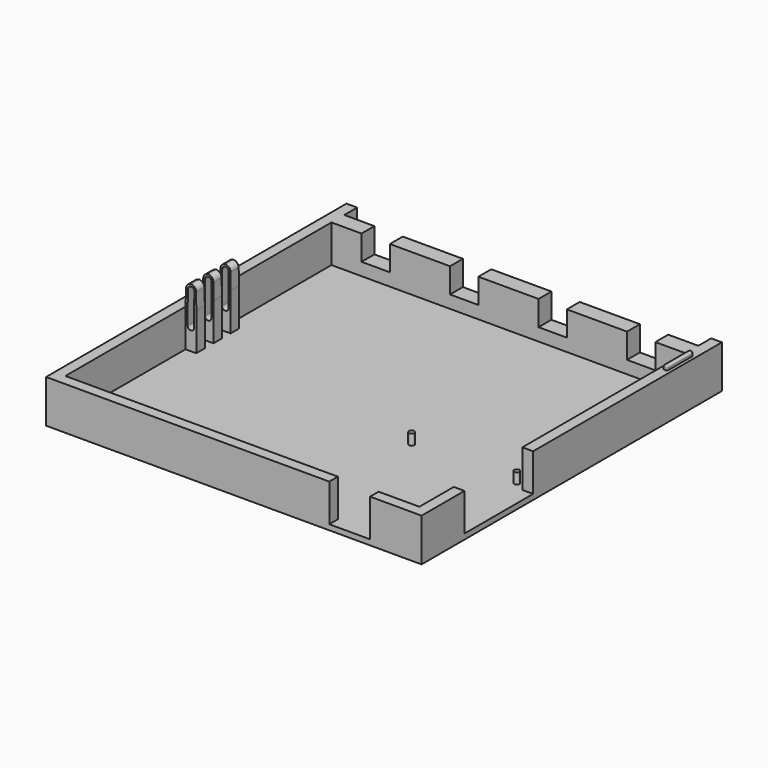
from build123d import *

# Parameters (mm, degrees)
F0_W           = 175
F0_H           = 175
F1_DEPTH       = 20
F2_W           = 165
F2_H           = 155
F3_DEPTH       = 17.5
F4_R           = 1.25
F5_DEPTH       = 5
F6_W           = 165
F6_H           = 7.5
F7_DEPTH       = 17.5
F8_W           = 13.2
F8_H           = 5.7
F9_DEPTH       = 8.5
F10_W          = 5
F10_H          = 5
F11_DEPTH      = 17.5
F11_DEPTH_BACK = 10
F11_TAPER_BACK = 1
F12_T1_DEPTH   = 16.9346144904
F12_T3_DEPTH   = 16.9346144904
F12_T5_DEPTH   = 16.9346144904
F14_DEPTH      = 25
F15_W          = 19
F15_H          = 17.6808023453
F15_W_2        = 32.2772479057
F15_H_2        = 40
F16_DEPTH      = 17.5
F17_W          = 13.2
F17_H          = 5.9
F18_DEPTH      = 8.5
F19_W          = 2
F19_H          = 15
F20_DEPTH      = 2
F21_R          = 0.99999
F22_R          = 0.5


# Not quite as in the source:
# - a fillet or chamfer that OpenCascade refuses, or shapes differently, is made with other operations: its cross-section is extruded or revolved along the edge and cut away or added
# - a fillet or chamfer is up to 0.001 mm smaller than in the source, because OpenCascade refuses the exact size


with BuildPart() as f1:
    # F0 (on Top) → F1 (new body)
    with BuildSketch(Plane.XY):
        Rectangle(F0_W, F0_H)
    extrude(amount=F1_DEPTH)

    # F2 (on face) → F3 (cut)
    with BuildSketch(Plane.XY.offset(20)):
        with Locations((0, -5)):
            Rectangle(F2_W, F2_H)
    extrude(amount=-F3_DEPTH, mode=Mode.SUBTRACT)

    # F4 (on face) → F5 (join)
    with BuildSketch(Plane.XY.offset(2.5)):
        with Locations((28.5, -77.5)):
            Circle(F4_R)
        with Locations((28.5, -19.5)):
            Circle(F4_R)
        with Locations((77.5, -77.5)):
            Circle(F4_R)
        with Locations((77.5, -19.5)):
            Circle(F4_R)
    extrude(amount=F5_DEPTH)

    # F6 (on face) → F7 (cut)
    with BuildSketch(Plane.XY.offset(20)):
        with Locations((0, 83.75)):
            Rectangle(F6_W, F6_H)
    extrude(amount=-F7_DEPTH, mode=Mode.SUBTRACT)

    # F8 (on face) → F9 (cut)
    with BuildSketch(Plane(origin=(0, 80, 0), x_dir=(-1, 0, 0), z_dir=(0, 1, 0))):
        with Locations((-61.875, 11.25)):
            Rectangle(F8_W, F8_H)
        with Locations((-20.625, 11.25)):
            Rectangle(F8_W, F8_H)
        with Locations((20.625, 11.25)):
            Rectangle(F8_W, F8_H)
        with Locations((61.875, 11.25)):
            Rectangle(F8_W, F8_H)
    extrude(amount=-F9_DEPTH, mode=Mode.SUBTRACT)

    # F10 (on face) → F11 (join, two sides)
    with BuildSketch(Plane.XY.offset(20)) as f11_sk:
        with Locations((-80, 0)):
            Rectangle(F10_W, F10_H)
        with Locations((-80, 10)):
            Rectangle(F10_W, F10_H)
        with Locations((-80, -10)):
            Rectangle(F10_W, F10_H)
    extrude(amount=-F11_DEPTH)
    extrude(f11_sk.sketch, amount=F11_DEPTH_BACK, taper=F11_TAPER_BACK)

    # F12: fillet of radius 2.5 on 6 edges, made by hand

    # F12_s2 → F12_t1 (cut)
    with BuildSketch(Plane.XZ.offset(-18.4673072452)):
        with BuildLine():
            ThreePointArc((-82.3683254308, 27.5436310161), (-81.6209793537, 29.2831261229), (-79.8687061929, 30))
            Line((-79.8687061929, 30), (-82.3254493507, 30))
            Line((-82.3254493507, 30), (-82.3683254308, 27.5436310161))
        make_face()
        with BuildLine():
            ThreePointArc((-80.1312938071, 30), (-78.3790206463, 29.2831261229), (-77.6316745692, 27.5436310161))
            Line((-77.6316745692, 27.5436310161), (-77.6745506493, 30))
            Line((-77.6745506493, 30), (-80.1312938071, 30))
        make_face()
    extrude(amount=F12_T1_DEPTH, mode=Mode.SUBTRACT)

    # F12_s4 → F12_t3 (cut)
    with BuildSketch(Plane.XZ.offset(-8.4673072452)):
        with BuildLine():
            ThreePointArc((-82.3683254308, 27.5436310161), (-81.6209793537, 29.2831261229), (-79.8687061929, 30))
            Line((-79.8687061929, 30), (-82.3254493507, 30))
            Line((-82.3254493507, 30), (-82.3683254308, 27.5436310161))
        make_face()
        with BuildLine():
            ThreePointArc((-80.1312938071, 30), (-78.3790206463, 29.2831261229), (-77.6316745692, 27.5436310161))
            Line((-77.6316745692, 27.5436310161), (-77.6745506493, 30))
            Line((-77.6745506493, 30), (-80.1312938071, 30))
        make_face()
    extrude(amount=F12_T3_DEPTH, mode=Mode.SUBTRACT)

    # F12_s6 → F12_t5 (cut)
    with BuildSketch(Plane.XZ.offset(1.5326927548)):
        with BuildLine():
            ThreePointArc((-82.3683254308, 27.5436310161), (-81.6209793537, 29.2831261229), (-79.8687061929, 30))
            Line((-79.8687061929, 30), (-82.3254493507, 30))
            Line((-82.3254493507, 30), (-82.3683254308, 27.5436310161))
        make_face()
        with BuildLine():
            ThreePointArc((-80.1312938071, 30), (-78.3790206463, 29.2831261229), (-77.6316745692, 27.5436310161))
            Line((-77.6316745692, 27.5436310161), (-77.6745506493, 30))
            Line((-77.6745506493, 30), (-80.1312938071, 30))
        make_face()
    extrude(amount=F12_T5_DEPTH, mode=Mode.SUBTRACT)

    # F13 (on face) → F14 (cut)
    with BuildSketch(Plane(origin=(0, 12.5, 0), x_dir=(-1, 0, 0), z_dir=(0, 1, 0))):
        with BuildLine():
            Line((81.5, 12.5), (81.5, 27.5))
            ThreePointArc((81.5, 27.5), (80, 29), (78.5, 27.5))
            Line((78.5, 27.5), (78.5, 12.5))
            ThreePointArc((78.5, 12.5), (80, 11), (81.5, 12.5))
        make_face()
    extrude(amount=-F14_DEPTH, mode=Mode.SUBTRACT)

    # F15 (on face) → F16 (cut)
    with BuildSketch(Plane.XY.offset(20)):
        with Locations((54, -82.5)):
            Rectangle(F15_W, F15_H)
        with Locations((82.5, -42.5)):
            Rectangle(F15_W_2, F15_H_2)
    extrude(amount=-F16_DEPTH, mode=Mode.SUBTRACT)

    # F17 (on face) → F18 (cut)
    with BuildSketch(Plane(origin=(0, 80, 0), x_dir=(-1, 0, 0), z_dir=(0, 1, 0))):
        with Locations((-61.875, 17.05)):
            Rectangle(F17_W, F17_H)
        with Locations((-20.625, 17.05)):
            Rectangle(F17_W, F17_H)
        with Locations((20.625, 17.05)):
            Rectangle(F17_W, F17_H)
        with Locations((61.875, 17.05)):
            Rectangle(F17_W, F17_H)
    extrude(amount=-F18_DEPTH, mode=Mode.SUBTRACT)

    # F19 (on face) → F20 (join)
    with BuildSketch(Plane.XY.offset(20)):
        with Locations((85, 65)):
            Rectangle(F19_W, F19_H)
    extrude(amount=F20_DEPTH)

    # F21 (radius 1 in the source; OpenCascade refuses exactly that, so slightly less here)
    f21_edges = [f1.edges().sort_by_distance(p)[0] for p in [
        (84, 65, 22),
        (86, 65, 22),
    ]]
    fillet(f21_edges, radius=F21_R)

    # F22
    f22_edges = [f1.edges().sort_by_distance(p)[0] for p in [
        (85.70711, 57.5, 21.70711),
        (85.70711, 72.5, 21.70711),
        (86, 57.5, 20.500005),
        (86, 72.5, 20.500005),
        (84, 57.5, 20.500005),
        (84.29289, 57.5, 21.70711),
        (85, 57.5, 22),
        (85, 72.5, 22),
        (84, 72.5, 20.500005),
        (84.29289, 72.5, 21.70711),
    ]]
    fillet(f22_edges, radius=F22_R)


solid = f1.part
